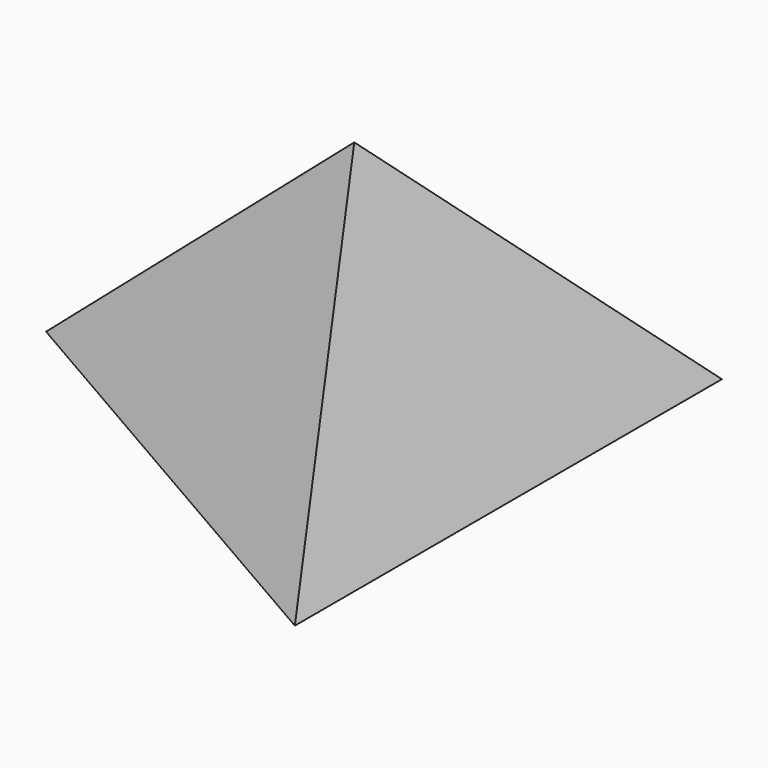
from build123d import *

# Parameters (mm, degrees)
F1_DEPTH = 19.05
F2_SIZE2 = 10.998513
F2_SIZE  = 19.04999


# Not quite as in the source:
# - a fillet or chamfer is up to 0.001 mm smaller than in the source, because OpenCascade refuses the exact size


with BuildPart() as f1:
    # F0 (on Top) → F1 (new body)
    with BuildSketch(Plane.XY):
        Polygon((10.9985226281, -19.05), (10.9985226281, 19.05), (-21.9970452561, 0), align=None)
    extrude(amount=F1_DEPTH)

    # F2 (size 19.05 and 10.9985226281 in the source; OpenCascade refuses exactly that, so slightly less here)
    f2_edges = [f1.edges().sort_by_distance(p)[0] for p in [
        (-5.499261, -9.525, 19.05),
        (-5.499261, 9.525, 19.05),
        (10.998523, 0, 19.05),
    ]]
    chamfer(f2_edges, length=F2_SIZE, length2=F2_SIZE2)


solid = f1.part
